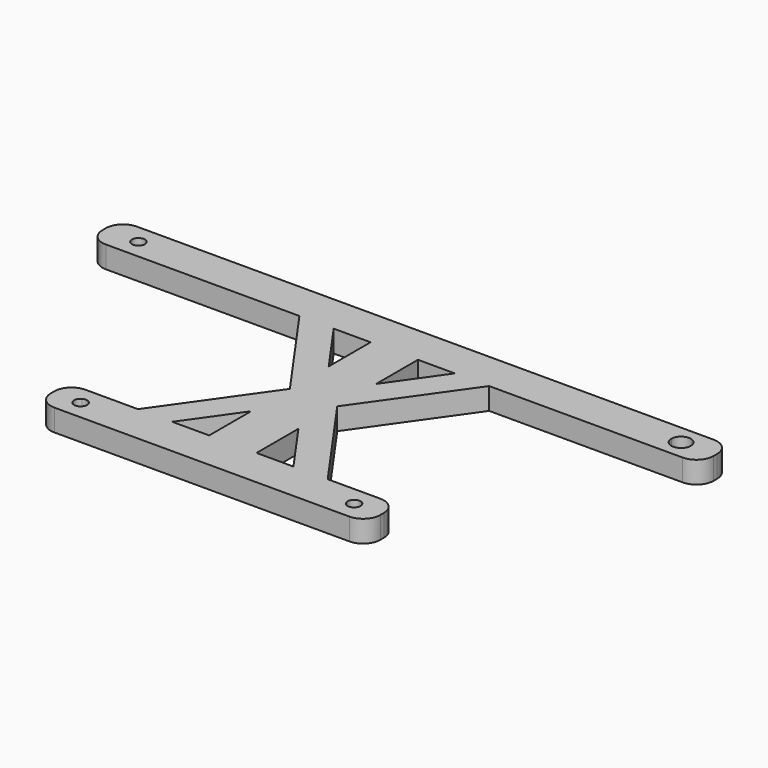
from build123d import *

# Parameters (mm, degrees)
F1_DEPTH = 5.08
F2_R     = 4


# Not quite as in the source:
# - a feature names something its author has since deleted; it is built from what else it names


with BuildPart() as f1:
    # F0 (on Top) → F1 (new body)
    with BuildSketch(Plane.XY):
        with BuildLine():
            Line((10.9156670719, 55.8519247654), (-50.5843329281, 55.8519247654))
            ThreePointArc((-50.5843329281, 55.8519247654), (-50.7903791398, 55.0931866065), (-51.3519110531, 54.5428952787))
            Line((-51.3519110531, 54.5428952787), (-49.566514597, 51.3519247654))
            Line((-49.566514597, 51.3519247654), (-11.1088099211, 51.3519247654))
            Line((-11.1088099211, 51.3519247654), (-3.1543997556, 51.3519247654))
            Line((-3.1543997556, 51.3519247654), (5.4156670719, 51.3519247654))
            Line((5.4156670719, 51.3519247654), (10.9156670719, 51.3519247654))
            Line((10.9156670719, 51.3519247654), (10.9156670719, 55.8519247654))
        make_face()
        with BuildLine():
            Line((-11.1088099211, 4.5), (-23.3521512592, 4.5))
            Line((-23.3521512592, 4.5), (-21.5667548031, 1.3090294867))
            ThreePointArc((-21.5667548031, 1.3090294867), (-20.0755947692, 1.2939537883), (-19.3343329281, 0))
            Line((-19.3343329281, 0), (10.9156670719, 0))
            Line((10.9156670719, 0), (10.9156670719, 4.5))
            Line((10.9156670719, 4.5), (5.4156670719, 4.5))
            Line((5.4156670719, 4.5), (-3.1543997556, 4.5))
            Line((-3.1543997556, 4.5), (-11.1088099211, 4.5))
        make_face()
        with BuildLine():
            ThreePointArc((-51.3519110531, 54.5428952787), (-53.3782867164, 56.6106629243), (-50.5843329281, 55.8519247654))
            Line((-50.5843329281, 55.8519247654), (10.9156670719, 55.8519247654))
            Line((10.9156670719, 55.8519247654), (71.6656670719, 55.8519247654))
            ThreePointArc((71.6656670719, 55.8519247654), (73.9156670719, 58.1019247654), (76.1656670719, 55.8519247654))
            ThreePointArc((76.1656670719, 55.8519247654), (75.0537743102, 53.910994083), (72.8170342594, 53.8883805354))
            Line((72.8170342594, 53.8883805354), (71.3978487408, 51.3519247654))
            Line((71.3978487408, 51.3519247654), (81.8841302488, 51.3519247654))
            Line((81.8841302488, 51.3519247654), (81.8841302488, 60.3519247654))
            Line((81.8841302488, 60.3519247654), (-60.052796105, 60.3519247654))
            Line((-60.052796105, 60.3519247654), (-60.052796105, 51.3519247654))
            Line((-60.052796105, 51.3519247654), (-49.566514597, 51.3519247654))
            Line((-49.566514597, 51.3519247654), (-51.3519110531, 54.5428952787))
        make_face()
        with BuildLine():
            Line((-21.5667548031, 1.3090294867), (-23.3521512592, 4.5))
            Line((-23.3521512592, 4.5), (-27.3365851734, 4.5))
            Line((-27.3365851734, 4.5), (-27.3365851734, -4.5))
            Line((-27.3365851734, -4.5), (49.1679193172, -4.5))
            Line((49.1679193172, -4.5), (49.1679193172, 4.5))
            Line((49.1679193172, 4.5), (45.183485403, 4.5))
            Line((45.183485403, 4.5), (43.3980889469, 1.3090294867))
            ThreePointArc((43.3980889469, 1.3090294867), (43.9596208602, 0.7587381589), (44.1656670719, 0))
            ThreePointArc((44.1656670719, 0), (42.6656670719, -1.5), (41.1656670719, 0))
            Line((41.1656670719, 0), (10.9156670719, 0))
            Line((10.9156670719, 0), (-19.3343329281, 0))
            ThreePointArc((-19.3343329281, 0), (-21.593071087, -1.2939537883), (-21.5667548031, 1.3090294867))
        make_face()
        with BuildLine():
            Line((16.4156670719, 4.5), (10.9156670719, 4.5))
            Line((10.9156670719, 4.5), (10.9156670719, 0))
            Line((10.9156670719, 0), (41.1656670719, 0))
            ThreePointArc((41.1656670719, 0), (41.906928913, 1.2939537883), (43.3980889469, 1.3090294867))
            Line((43.3980889469, 1.3090294867), (45.183485403, 4.5))
            Line((45.183485403, 4.5), (32.9401440649, 4.5))
            Line((32.9401440649, 4.5), (24.9857338994, 4.5))
            Line((24.9857338994, 4.5), (16.4156670719, 4.5))
        make_face()
        with BuildLine():
            Line((71.6656670719, 55.8519247654), (10.9156670719, 55.8519247654))
            Line((10.9156670719, 55.8519247654), (10.9156670719, 51.3519247654))
            Line((10.9156670719, 51.3519247654), (16.4156670719, 51.3519247654))
            Line((16.4156670719, 51.3519247654), (24.9857338994, 51.3519247654))
            Line((24.9857338994, 51.3519247654), (32.9401440649, 51.3519247654))
            Line((32.9401440649, 51.3519247654), (71.3978487408, 51.3519247654))
            Line((71.3978487408, 51.3519247654), (72.8170342594, 53.8883805354))
            ThreePointArc((72.8170342594, 53.8883805354), (71.9747363894, 54.7138175271), (71.6656670719, 55.8519247654))
        make_face()
        Polygon((10.9156670719, 27.9259623827), (10.9156670719, 51.3519247654), (5.4156670719, 51.3519247654), (5.4156670719, 39.2025500407), (5.4156670719, 27.9259623827), align=None)
        Polygon((10.9156670719, 4.5), (10.9156670719, 27.9259623827), (5.4156670719, 27.9259623827), (5.4156670719, 16.6493747247), (5.4156670719, 4.5), align=None)
        Polygon((16.4156670719, 51.3519247654), (10.9156670719, 51.3519247654), (10.9156670719, 27.9259623827), (16.4156670719, 27.9259623827), (16.4156670719, 39.2025500407), align=None)
        Polygon((16.4156670719, 27.9259623827), (10.9156670719, 27.9259623827), (10.9156670719, 4.5), (16.4156670719, 4.5), (16.4156670719, 16.6493747247), align=None)
        Polygon((-3.1543997556, 51.3519247654), (-11.1088099211, 51.3519247654), (5.4156670719, 27.9259623827), (5.4156670719, 39.2025500407), align=None)
        Polygon((5.4156670719, 27.9259623827), (-11.1088099211, 4.5), (-3.1543997556, 4.5), (5.4156670719, 16.6493747247), align=None)
        Polygon((32.9401440649, 4.5), (16.4156670719, 27.9259623827), (16.4156670719, 16.6493747247), (24.9857338994, 4.5), align=None)
        Polygon((16.4156670719, 39.2025500407), (16.4156670719, 27.9259623827), (32.9401440649, 51.3519247654), (24.9857338994, 51.3519247654), align=None)
    extrude(amount=F1_DEPTH)

    # F2
    f2_edges = [f1.edges().sort_by_distance(p)[0] for p in [
        (-60.052796, 60.351925, 2.54),
        (-60.052796, 51.351925, 2.54),
        (81.88413, 60.351925, 2.54),
        (81.88413, 51.351925, 2.54),
        (49.167919, 4.5, 2.54),
        (49.167919, -4.5, 2.54),
        (-27.336585, 4.5, 2.54),
        (-27.336585, -4.5, 2.54),
    ]]
    fillet(f2_edges, radius=F2_R)


solid = f1.part
